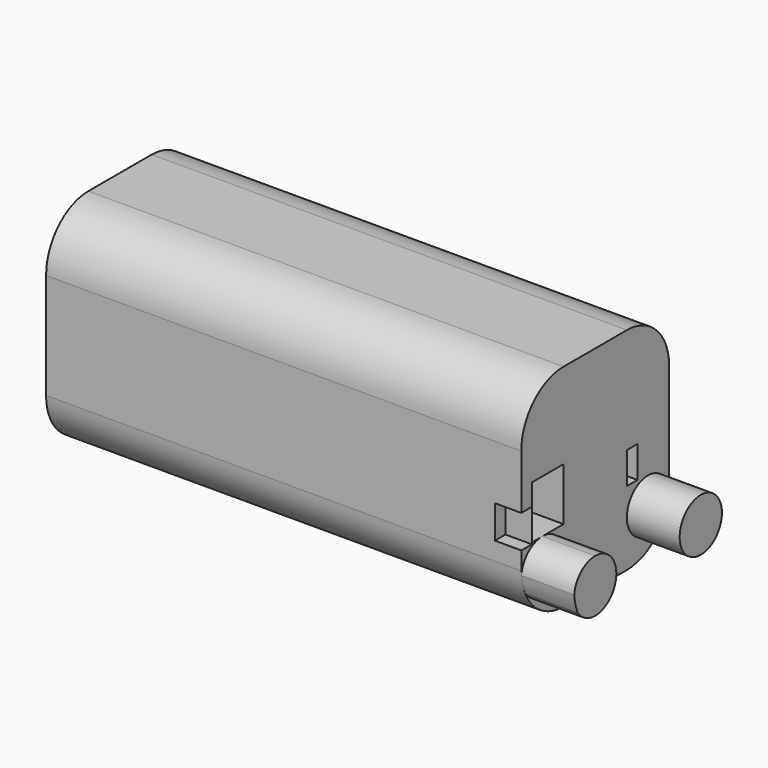
from build123d import *

# Parameters (mm, degrees)
F0_W      = 45.72
F0_H      = 17.78
F1_DEPTH  = 20.32
F2_R      = 5.08
F3_W      = 3.7871776995
F3_H      = 5.08
F3_W_2    = 3.7677848834
F4_DEPTH  = 5.08
F9_W      = 1.27
F9_H      = 3.175
F9_H_2    = 3.048
F10_DEPTH = 2.54
F12_DEPTH = 5.08


# Not quite as in the source:
# - the program builds the solid bodies; features that only make, move or delete a surface that nothing else refers to are left out


with BuildPart() as f1:
    # F0 (on Top) → F1 (new body)
    with BuildSketch(Plane.XY):
        with Locations((22.86, 8.89)):
            Rectangle(F0_W, F0_H)
    extrude(amount=F1_DEPTH)

    # F2
    f2_edges = [f1.edges().sort_by_distance(p)[0] for p in [
        (22.86, 17.78, 20.32),
        (22.86, 0, 20.32),
        (22.86, 17.78, 0),
        (22.86, 0, 0),
    ]]
    fillet(f2_edges, radius=F2_R)

    # F3 (on face) → F4 (cut)
    with BuildSketch(Plane.YZ.offset(45.72)):
        with Locations((3.1864111502, 9.525)):
            Rectangle(F3_W, F3_H)
        with Locations((22.2461075583, 9.525)):
            Rectangle(F3_W_2, F3_H)
    extrude(amount=-F4_DEPTH, mode=Mode.SUBTRACT)

    # F9 (on face) → F10 (cut)
    with BuildSketch(Plane.YZ.offset(45.72)):
        with Locations((0.635, 8.4111910738)):
            Rectangle(F9_W, F9_H)
        with Locations((13.335, 8.636)):
            Rectangle(F9_W, F9_H_2)
    extrude(amount=-F10_DEPTH, mode=Mode.SUBTRACT)


with BuildPart() as f12:
    # F11 (on face) → F12 (new body)
    with BuildSketch(Plane.YZ.offset(45.72)):
        with BuildLine():
            ThreePointArc((0.4345907815, 3.0241368741), (3.2829201118, 2.0160764303), (5.08, 4.445))
            ThreePointArc((5.08, 4.445), (4.3360512242, 6.2410512242), (2.54, 6.985))
            ThreePointArc((2.54, 6.985), (0.839444466, 6.3317196071), (0.0136445126, 4.7079219494))
            ThreePointArc((0.0136445126, 4.7079219494), (0.1516760993, 3.8479190248), (0.4345907815, 3.0241368741))
        make_face()
    extrude(amount=F12_DEPTH)


with BuildPart() as f12b:
    # F11 (on face) → F12, piece 2 (new body)
    with BuildSketch(Plane.YZ.offset(45.72)):
        with BuildLine():
            ThreePointArc((17.7663554874, 4.7079219494), (17.6283239007, 3.8479190248), (17.3454092185, 3.0241368741))
            ThreePointArc((17.3454092185, 3.0241368741), (17.6689235697, 3.7020798882), (17.78, 4.445))
            ThreePointArc((17.78, 4.445), (17.7765865782, 4.5766378785), (17.7663554874, 4.7079219494))
        make_face()
        with BuildLine():
            ThreePointArc((17.7663554874, 4.7079219494), (12.7758380496, 5.0610404876), (17.3454092185, 3.0241368741))
            ThreePointArc((17.3454092185, 3.0241368741), (17.6283239007, 3.8479190248), (17.7663554874, 4.7079219494))
        make_face()
    extrude(amount=F12_DEPTH)


solid = Compound([f1.part, f12.part, f12b.part])
